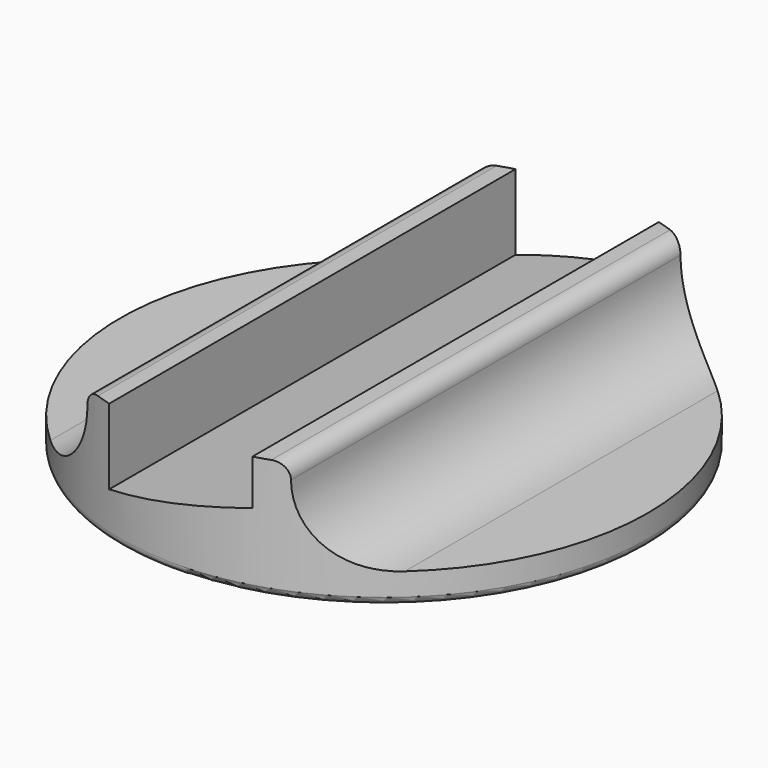
from build123d import *

# Parameters (mm, degrees)
F0_R     = 17.5
F1_DEPTH = 2
F3_DEPTH = 20
F4_DEPTH = 6.001
F5_DEPTH = 6.001
F6_R     = 5
F7_R     = 0.99999
F8_R     = 0.5


# Not quite as in the source:
# - a fillet or chamfer is up to 0.001 mm smaller than in the source, because OpenCascade refuses the exact size


with BuildPart() as f1:
    # F0 (on Top) → F1 (new body)
    with BuildSketch(Plane.XY):
        Circle(F0_R)
    extrude(amount=F1_DEPTH)

    # F2 (on Front) → F3 (join, symmetric)
    with BuildSketch(Plane.XZ):
        Polygon((-6.75, 8), (-6.75, 2), (6.75, 2), (6.75, 8), (4.75, 8), (4.75, 5), (-4.75, 3), (-4.75, 8), align=None)
    extrude(amount=F3_DEPTH, both=True)

    # F4 (cut, through all): a face of the model
    f4_faces = [f1.faces().sort_by_distance(p)[0] for p in [
        (0, -18.5005607704, 2),
    ]]
    extrude(f4_faces, amount=-F4_DEPTH, mode=Mode.SUBTRACT)

    # F5 (cut, through all): a face of the model
    f5_faces = [f1.faces().sort_by_distance(p)[0] for p in [
        (0, 18.5005607704, 2),
    ]]
    extrude(f5_faces, amount=-F5_DEPTH, mode=Mode.SUBTRACT)

    # F6
    f6_edges = [f1.edges().sort_by_distance(p)[0] for p in [
        (-6.75, 0, 2),
        (6.75, 0, 2),
    ]]
    fillet(f6_edges, radius=F6_R)

    # F7 (radius 1 in the source; OpenCascade refuses exactly that, so slightly less here)
    f7_edges = [f1.edges().sort_by_distance(p)[0] for p in [
        (-6.75, 0, 8),
        (6.75, 0, 8),
    ]]
    fillet(f7_edges, radius=F7_R)

    # F8
    f8_edges = [f1.edges().sort_by_distance(p)[0] for p in [
        (-17.5, 0, 0),
    ]]
    fillet(f8_edges, radius=F8_R)


solid = f1.part
